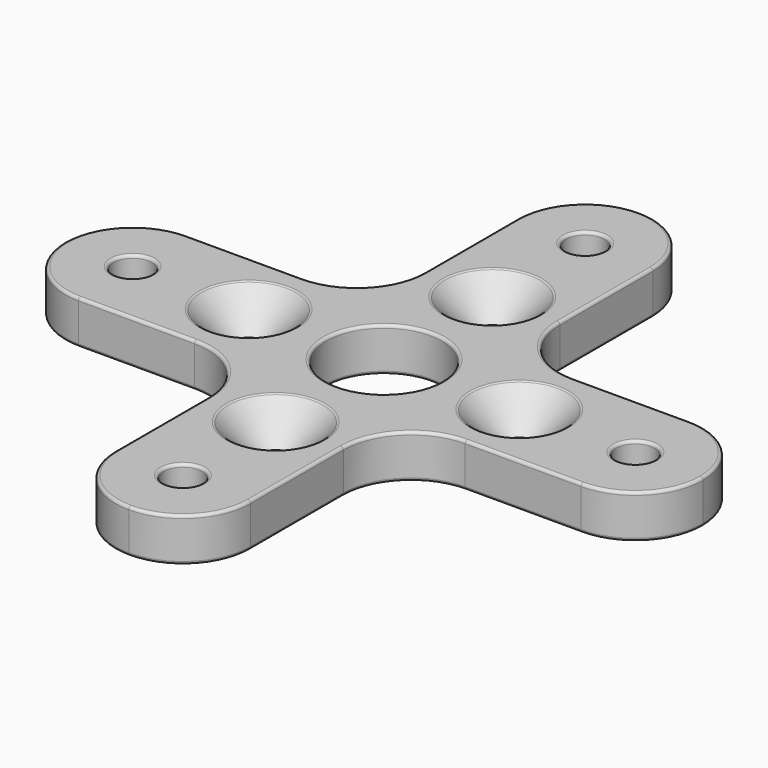
from build123d import *

# Parameters (mm, degrees)
F0_R     = 1
F0_R_2   = 0.8
F0_R_3   = 3
F1_DEPTH = 2.25
F2_R     = 3.49999
F3_SIZE  = 1.7
F4_R     = 0.15


# Not quite as in the source:
# - a fillet or chamfer is up to 0.001 mm smaller than in the source, because OpenCascade refuses the exact size


with BuildPart() as f1:
    # F0 (on Top) → F1 (new body)
    with BuildSketch(Plane.XY):
        Polygon((-25.8403990492, -37.8702705037), (-18.8403990492, -37.8702705037), (-18.8403990492, -24.8702705037), (-5.8403990492, -24.8702705037), (-5.8403990492, -17.8702705037), (-18.8403990492, -17.8702705037), (-18.8403990492, -4.8702705037), (-25.8403990492, -4.8702705037), (-25.8403990492, -17.8702705037), (-38.8403990492, -17.8702705037), (-38.8403990492, -24.8702705037), (-25.8403990492, -24.8702705037), align=None)
        with Locations((-22.3403990492, -34.3702705037)):
            Circle(F0_R, mode=Mode.SUBTRACT)
        with Locations((-22.3403990492, -28.3702705037)):
            Circle(F0_R_2, mode=Mode.SUBTRACT)
        with Locations((-35.3403990492, -21.3702705037)):
            Circle(F0_R, mode=Mode.SUBTRACT)
        with Locations((-29.3403990492, -21.3702705037)):
            Circle(F0_R_2, mode=Mode.SUBTRACT)
        with Locations((-22.3403990492, -21.3702705037)):
            Circle(F0_R_3, mode=Mode.SUBTRACT)
        with Locations((-15.3403990492, -21.3702705037)):
            Circle(F0_R_2, mode=Mode.SUBTRACT)
        with Locations((-22.3403990492, -14.3702705037)):
            Circle(F0_R_2, mode=Mode.SUBTRACT)
        with Locations((-9.3403990492, -21.3702705037)):
            Circle(F0_R, mode=Mode.SUBTRACT)
        with Locations((-22.3403990492, -8.3702705037)):
            Circle(F0_R, mode=Mode.SUBTRACT)
    extrude(amount=F1_DEPTH)

    # F2 (radius 3.5 in the source; OpenCascade refuses exactly that, so slightly less here)
    f2_edges = [f1.edges().sort_by_distance(p)[0] for p in [
        (-25.840399, -4.870271, 1.125),
        (-18.840399, -4.870271, 1.125),
        (-5.840399, -17.870271, 1.125),
        (-5.840399, -24.870271, 1.125),
        (-18.840399, -37.870271, 1.125),
        (-25.840399, -37.870271, 1.125),
        (-38.840399, -24.870271, 1.125),
        (-38.840399, -17.870271, 1.125),
        (-25.840399, -24.870271, 1.125),
        (-18.840399, -24.870271, 1.125),
        (-18.840399, -17.870271, 1.125),
        (-25.840399, -17.870271, 1.125),
    ]]
    fillet(f2_edges, radius=F2_R)

    # F3
    f3_edges = [f1.edges().sort_by_distance(p)[0] for p in [
        (-23.140399, -14.370271, 2.25),
        (-16.140399, -21.370271, 2.25),
        (-23.140399, -28.370271, 2.25),
        (-30.140399, -21.370271, 2.25),
    ]]
    chamfer(f3_edges, length=F3_SIZE)

    # F4
    f4_edges = [f1.edges().sort_by_distance(p)[0] for p in [
        (-24.840399, -14.370271, 2.25),
        (-25.840399, -11.370271, 2.25),
        (-24.815276, -5.895394, 2.25),
        (-26.865522, -16.845147, 2.25),
        (-22.340399, -4.870271, 2.25),
        (-32.340399, -17.870271, 2.25),
        (-19.865522, -5.895394, 2.25),
        (-37.815276, -18.895394, 2.25),
        (-18.840399, -11.370271, 2.25),
        (-38.840399, -21.370271, 2.25),
        (-17.815276, -16.845147, 2.25),
        (-37.815276, -23.845147, 2.25),
        (-12.340399, -17.870271, 2.25),
        (-32.340399, -24.870271, 2.25),
        (-6.865522, -18.895394, 2.25),
        (-26.865522, -25.895394, 2.25),
        (-5.840399, -21.370271, 2.25),
        (-25.840399, -31.370271, 2.25),
        (-6.865522, -23.845147, 2.25),
        (-24.815276, -36.845147, 2.25),
        (-12.340399, -24.870271, 2.25),
        (-22.340399, -37.870271, 2.25),
        (-17.815276, -25.895394, 2.25),
        (-19.865522, -36.845147, 2.25),
        (-18.840399, -31.370271, 2.25),
        (-23.340399, -34.370271, 2.25),
        (-36.340399, -21.370271, 2.25),
        (-25.340399, -21.370271, 2.25),
        (-10.340399, -21.370271, 2.25),
        (-23.340399, -8.370271, 2.25),
        (-17.840399, -21.370271, 2.25),
        (-24.840399, -28.370271, 2.25),
        (-31.840399, -21.370271, 2.25),
        (-25.840399, -11.370271, 0),
        (-24.815276, -5.895394, 0),
        (-26.865522, -16.845147, 0),
        (-22.340399, -4.870271, 0),
        (-32.340399, -17.870271, 0),
        (-19.865522, -5.895394, 0),
        (-37.815276, -18.895394, 0),
        (-18.840399, -11.370271, 0),
        (-38.840399, -21.370271, 0),
        (-17.815276, -16.845147, 0),
        (-37.815276, -23.845147, 0),
        (-12.340399, -17.870271, 0),
        (-32.340399, -24.870271, 0),
        (-6.865522, -18.895394, 0),
        (-26.865522, -25.895394, 0),
        (-5.840399, -21.370271, 0),
        (-25.840399, -31.370271, 0),
        (-6.865522, -23.845147, 0),
        (-24.815276, -36.845147, 0),
        (-12.340399, -24.870271, 0),
        (-22.340399, -37.870271, 0),
        (-17.815276, -25.895394, 0),
        (-19.865522, -36.845147, 0),
        (-18.840399, -31.370271, 0),
        (-23.340399, -34.370271, 0),
        (-23.140399, -28.370271, 0),
        (-36.340399, -21.370271, 0),
        (-30.140399, -21.370271, 0),
        (-25.340399, -21.370271, 0),
        (-16.140399, -21.370271, 0),
        (-23.140399, -14.370271, 0),
        (-10.340399, -21.370271, 0),
        (-23.340399, -8.370271, 0),
    ]]
    fillet(f4_edges, radius=F4_R)


solid = f1.part
